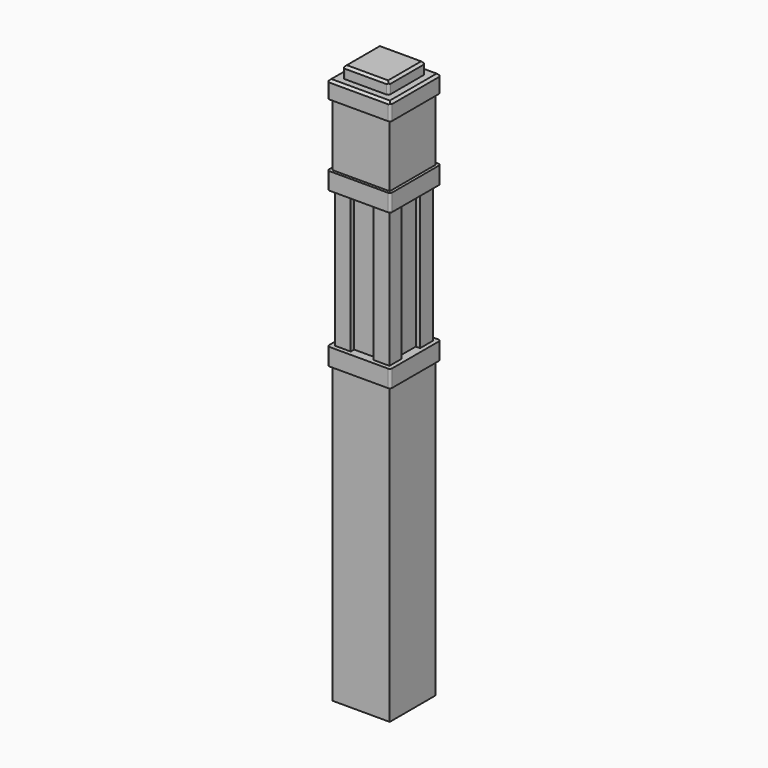
from build123d import *

# Parameters (mm, degrees)
F0_W      = 88.9
F0_H      = 88.9
F1_DEPTH  = 1193.8
F3_DEPTH  = 673.1
F4_W      = 139.7
F4_H      = 139.7
F4_W_2    = 127
F4_H_2    = 127
F5_DEPTH  = 19.05
F6_W      = 139.7
F6_H      = 139.7
F6_W_2    = 91.44
F6_H_2    = 91.44
F7_DEPTH  = 19.05
F8_W      = 101.6
F8_H      = 101.6
F8_W_2    = 88.9
F8_H_2    = 88.9
F9_DEPTH  = 304.8
F10_W     = 139.7
F10_H     = 139.7
F10_W_2   = 88.9
F10_H_2   = 88.9
F11_DEPTH = 19.05
F12_W     = 139.7
F12_H     = 139.7
F12_W_2   = 127
F12_H_2   = 127
F13_DEPTH = 19.05
F14_W     = 127
F14_H     = 127
F14_W_2   = 88.9
F14_H_2   = 88.9
F15_DEPTH = 177.8
F16_W     = 120.65
F16_H     = 120.65
F16_W_2   = 101.6
F16_H_2   = 101.6
F17_DEPTH = 304.8
F18_W     = 9.525
F18_H     = 50.8
F18_W_2   = 50.8
F18_H_2   = 9.525
F19_DEPTH = 304.8
F20_W     = 139.7
F20_H     = 139.7
F20_W_2   = 127
F20_H_2   = 127
F21_DEPTH = 19.05
F22_W     = 139.7
F22_H     = 139.7
F23_DEPTH = 19.05
F24_W     = 101.6
F24_H     = 101.6
F25_DEPTH = 25.4
F26_SIZE  = 5.08
F27_R     = 5.08
F27_2_R   = 5.08
F27_3_R   = 5.08


with BuildPart() as f1:
    # F0 (on Top) → F1 (new body)
    with BuildSketch(Plane.XY):
        Rectangle(F0_W, F0_H)
    extrude(amount=F1_DEPTH)


with BuildPart() as f3:
    # F2 (on face) → F3 (new body)
    with BuildSketch(Plane(origin=(0, 0, 0), x_dir=(1, 0, 0), z_dir=(0, 0, -1))):
        Polygon((-44.45, 44.45), (-63.5, 63.5), (-63.5, -63.5), (-44.45, -44.45), align=None)
        Polygon((63.5, 63.5), (-63.5, 63.5), (-44.45, 44.45), (44.45, 44.45), align=None)
        Polygon((63.5, -63.5), (63.5, 63.5), (44.45, 44.45), (44.45, -44.45), align=None)
        Polygon((-44.45, -44.45), (-63.5, -63.5), (63.5, -63.5), (44.45, -44.45), align=None)
    extrude(amount=-F3_DEPTH)


with BuildPart() as f5:
    # F4 (on face) → F5 (new body)
    with BuildSketch(Plane.XY.offset(673.1)):
        Rectangle(F4_W, F4_H)
        Rectangle(F4_W_2, F4_H_2, mode=Mode.SUBTRACT)
    extrude(amount=-F5_DEPTH)

    # F6 (on face) → F7 (join)
    with BuildSketch(Plane.XY.offset(673.1)):
        Rectangle(F6_W, F6_H)
        Rectangle(F6_W_2, F6_H_2, mode=Mode.SUBTRACT)
    extrude(amount=F7_DEPTH)

    # F27
    f27_edges = [f5.edges().sort_by_distance(p)[0] for p in [
        (69.85, 69.85, 673.1),
        (69.85, -69.85, 673.1),
        (-69.85, -69.85, 673.1),
        (-69.85, 69.85, 673.1),
    ]]
    fillet(f27_edges, radius=F27_R)


with BuildPart() as f9:
    # F8 (on face) → F9 (new body)
    with BuildSketch(Plane.XY.offset(692.15)):
        Rectangle(F8_W, F8_H)
        Rectangle(F8_W_2, F8_H_2, mode=Mode.SUBTRACT)
    extrude(amount=F9_DEPTH)


with BuildPart() as f11:
    # F10 (on face) → F11 (new body)
    with BuildSketch(Plane.XY.offset(996.95)):
        Rectangle(F10_W, F10_H)
        Rectangle(F10_W_2, F10_H_2, mode=Mode.SUBTRACT)
    extrude(amount=F11_DEPTH)

    # F12 (on face) → F13 (join)
    with BuildSketch(Plane.XY.offset(1016)):
        Rectangle(F12_W, F12_H)
        Rectangle(F12_W_2, F12_H_2, mode=Mode.SUBTRACT)
    extrude(amount=F13_DEPTH)

    # F27#2
    f27_2_edges = [f11.edges().sort_by_distance(p)[0] for p in [
        (-69.85, -69.85, 1016),
        (69.85, -69.85, 1016),
        (-69.85, 69.85, 1016),
        (69.85, 69.85, 1016),
    ]]
    fillet(f27_2_edges, radius=F27_2_R)


with BuildPart() as f15:
    # F14 (on face) → F15 (new body)
    with BuildSketch(Plane.XY.offset(1016)):
        Rectangle(F14_W, F14_H)
        Rectangle(F14_W_2, F14_H_2, mode=Mode.SUBTRACT)
    extrude(amount=F15_DEPTH)


with BuildPart() as f17:
    # F16 (on face) → F17 (new body)
    with BuildSketch(Plane.XY.offset(692.15)):
        Rectangle(F16_W, F16_H)
        Rectangle(F16_W_2, F16_H_2, mode=Mode.SUBTRACT)
    extrude(amount=F17_DEPTH)

    # F18 (on face) → F19 (cut)
    with BuildSketch(Plane.XY.offset(996.95)):
        with Locations((-55.5625, -0.8699878395)):
            Rectangle(F18_W, F18_H)
        with Locations((55.5625, -0.8699878395)):
            Rectangle(F18_W, F18_H)
        with Locations((-0.0076036245, 55.5625)):
            Rectangle(F18_W_2, F18_H_2)
        with Locations((-0.0076036245, -55.5625)):
            Rectangle(F18_W_2, F18_H_2)
    extrude(amount=-F19_DEPTH, mode=Mode.SUBTRACT)


with BuildPart() as f21:
    # F20 (on face) → F21 (new body)
    with BuildSketch(Plane.XY.offset(1193.8)):
        Rectangle(F20_W, F20_H)
        Rectangle(F20_W_2, F20_H_2, mode=Mode.SUBTRACT)
    extrude(amount=-F21_DEPTH)

    # F22 (on face) → F23 (join)
    with BuildSketch(Plane.XY.offset(1193.8)):
        Rectangle(F22_W, F22_H)
    extrude(amount=F23_DEPTH)

    # F24 (on face) → F25 (join)
    with BuildSketch(Plane.XY.offset(1212.85)):
        Rectangle(F24_W, F24_H)
    extrude(amount=F25_DEPTH)

    # F26
    f26_edges = [f21.edges().sort_by_distance(p)[0] for p in [
        (0, 50.8, 1238.25),
        (-50.8, 0, 1238.25),
        (0, -50.8, 1238.25),
        (50.8, 0, 1238.25),
        (69.85, 0, 1212.85),
        (0, -69.85, 1212.85),
        (-69.85, 0, 1212.85),
        (0, 69.85, 1212.85),
    ]]
    chamfer(f26_edges, length=F26_SIZE)

    # F27#3
    f27_3_edges = [f21.edges().sort_by_distance(p)[0] for p in [
        (69.85, 69.85, 1191.26),
        (50.8, 50.8, 1223.01),
        (69.85, -69.85, 1191.26),
        (50.8, -50.8, 1223.01),
        (-69.85, -69.85, 1191.26),
        (-50.8, -50.8, 1223.01),
        (-69.85, 69.85, 1191.26),
        (-50.8, 50.8, 1223.01),
    ]]
    fillet(f27_3_edges, radius=F27_3_R)


solid = Compound([f1.part, f3.part, f5.part, f9.part, f11.part, f15.part, f17.part, f21.part])
